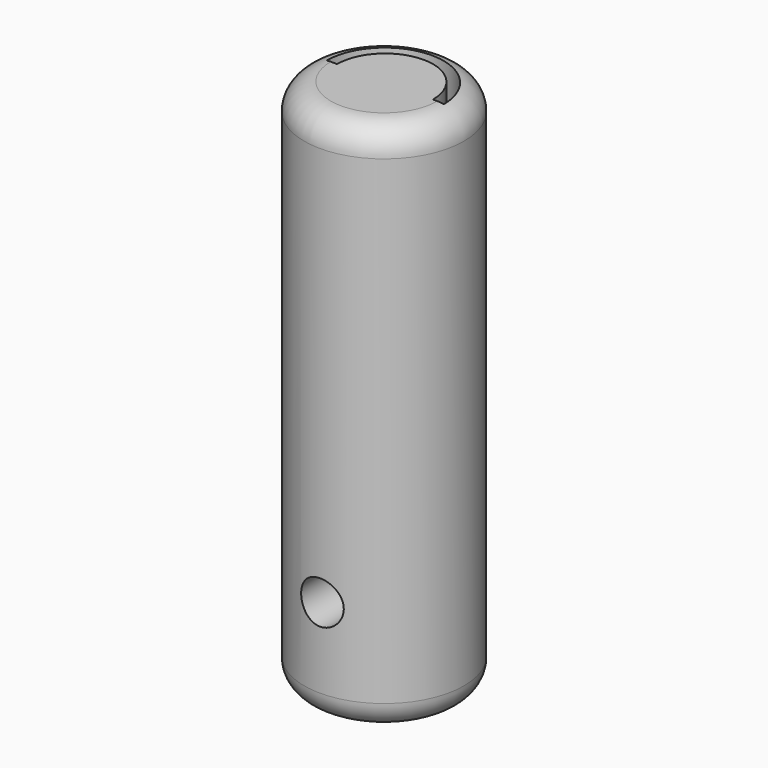
from build123d import *

# Parameters (mm, degrees)
F0_R          = 15
F1_DEPTH      = 100
F3_DEPTH      = 40
F5_R          = 4
F6_DEPTH      = 25
F6_DEPTH_BACK = 25


# Not quite as in the source:
# - a fillet or chamfer that OpenCascade refuses, or shapes differently, is made with other operations: its cross-section is extruded or revolved along the edge and cut away or added


with BuildPart() as f1:
    # F0 (on Top) → F1 (new body)
    with BuildSketch(Plane.XY):
        Circle(F0_R)
    extrude(amount=F1_DEPTH)

    # F2 (on face) → F3 (cut)
    with BuildSketch(Plane.XY.offset(100)):
        with BuildLine():
            Line((9.1818189363, 0), (11.1818189363, 0))
            ThreePointArc((11.1818189363, 0), (0.1818189363, 11), (-10.8181810637, 0))
            Line((-10.8181810637, 0), (-8.8181810637, 0))
            ThreePointArc((-8.8181810637, 0), (0.1818189363, 9), (9.1818189363, 0))
        make_face()
    extrude(amount=-F3_DEPTH, mode=Mode.SUBTRACT)

    # F4: fillet of radius 5 on 2 edges, made by hand

    # F4_s1 → F4_t2 (revolve, cut)
    with BuildSketch(Plane.XZ):
        with BuildLine():
            ThreePointArc((15, 95), (13.5355339059, 98.5355339059), (10, 100))
            Line((10, 100), (15, 100))
            Line((15, 100), (15, 95))
        make_face()
    revolve(axis=Axis((0, 0, 100), (0, 0, 1)), mode=Mode.SUBTRACT)

    # F4_s3 → F4_t4 (revolve, cut)
    with BuildSketch(Plane.XZ):
        with BuildLine():
            ThreePointArc((15, 5), (13.5355339059, 1.4644660941), (10, 0))
            Line((10, 0), (15, 0))
            Line((15, 0), (15, 5))
        make_face()
    revolve(axis=Axis((0, 0, 0), (0, 0, 1)), mode=Mode.SUBTRACT)

    # F5 (on Front) → F6 (cut, two sides)
    with BuildSketch(Plane.XZ) as f6_sk:
        with Locations((0, 20)):
            Circle(F5_R)
    extrude(amount=-F6_DEPTH, mode=Mode.SUBTRACT)
    extrude(f6_sk.sketch, amount=F6_DEPTH_BACK, mode=Mode.SUBTRACT)


solid = f1.part
